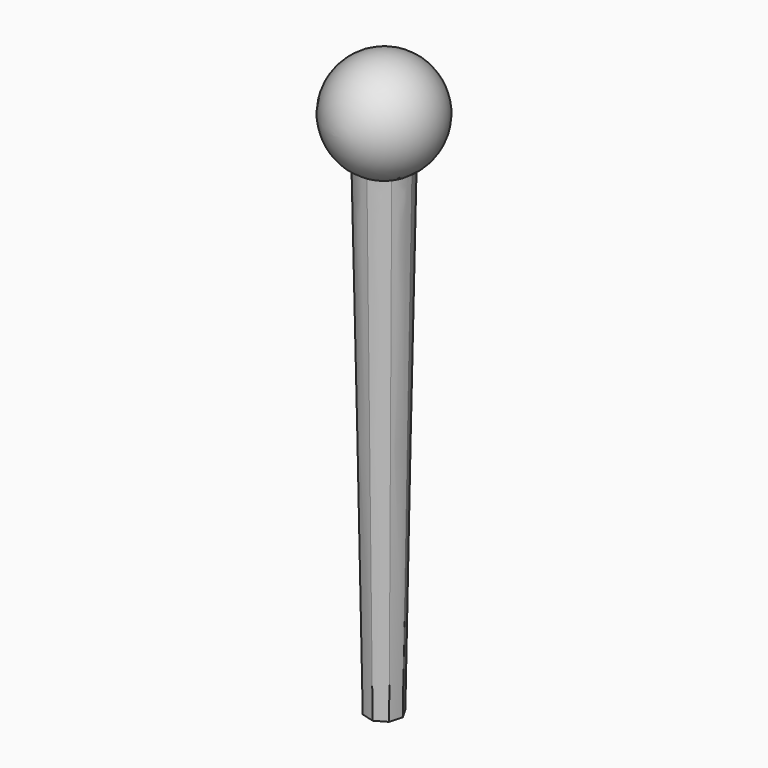
from build123d import *


# Not quite as in the source:
# - the arcs of a loft's sections are written as splines that run evenly, so that the points pair up as in the source's solid


with BuildPart() as f3:
    # F2 (on offset) → F3 section 0
    with BuildSketch(Plane.XY.offset(500)):
        with BuildLine():
            add(Edge.make_bspline(
                [(3.1036920521, -24.8065937937), (4.7272798193, -24.6034576239), (6.3308207683, -24.2404209935), (9.4363429336, -23.2084625424), (10.9382473598, -22.5395662389), (13.782772681, -20.9215792608), (15.1253232396, -19.972528594), (17.5995382038, -17.8306914211), (18.7311414296, -16.6379578761), (19.7355523864, -15.3462689929)],
                knots=[0, 0, 0, 0, 0.25, 0.25, 0.5, 0.5, 0.75, 0.75, 1, 1, 1, 1], degree=3))
            add(Edge.make_bspline(
                [(19.7355523864, -15.3462689929), (20.7399633433, -14.0545801097), (21.617132359, -12.6639997676), (23.0833633226, -9.7383591666), (23.6723890149, -8.2033712501), (24.5396825947, -5.0478985421), (24.8179290366, -3.427491776), (25.0529556268, -0.1634500075), (25.0097299635, 1.480104285), (24.8065937937, 3.1036920521)],
                knots=[0, 0, 0, 0, 0.25, 0.25, 0.5, 0.5, 0.75, 0.75, 1, 1, 1, 1], degree=3))
            add(Edge.make_bspline(
                [(24.8065937937, 3.1036920521), (24.6034576239, 4.7272798193), (24.2404209935, 6.3308207683), (23.2084625424, 9.4363429336), (22.5395662389, 10.9382473598), (20.9215792608, 13.782772681), (19.972528594, 15.1253232396), (17.8306914211, 17.5995382038), (16.6379578761, 18.7311414296), (15.3462689929, 19.7355523864)],
                knots=[0, 0, 0, 0, 0.25, 0.25, 0.5, 0.5, 0.75, 0.75, 1, 1, 1, 1], degree=3))
            add(Edge.make_bspline(
                [(15.3462689929, 19.7355523864), (14.0545801097, 20.7399633433), (12.6639997676, 21.617132359), (9.7383591666, 23.0833633226), (8.2033712501, 23.6723890149), (5.0478985421, 24.5396825947), (3.427491776, 24.8179290366), (0.1634500075, 25.0529556268), (-1.480104285, 25.0097299635), (-3.1036920521, 24.8065937937)],
                knots=[0, 0, 0, 0, 0.25, 0.25, 0.5, 0.5, 0.75, 0.75, 1, 1, 1, 1], degree=3))
            add(Edge.make_bspline(
                [(-3.1036920521, 24.8065937937), (-4.7272798193, 24.6034576239), (-6.3308207683, 24.2404209935), (-9.4363429336, 23.2084625424), (-10.9382473598, 22.5395662389), (-13.782772681, 20.9215792608), (-15.1253232396, 19.972528594), (-17.5995382038, 17.8306914211), (-18.7311414296, 16.6379578761), (-19.7355523864, 15.3462689929)],
                knots=[0, 0, 0, 0, 0.25, 0.25, 0.5, 0.5, 0.75, 0.75, 1, 1, 1, 1], degree=3))
            add(Edge.make_bspline(
                [(-19.7355523864, 15.3462689929), (-20.7399633433, 14.0545801097), (-21.617132359, 12.6639997676), (-23.0833633226, 9.7383591666), (-23.6723890149, 8.2033712501), (-24.5396825947, 5.0478985421), (-24.8179290366, 3.427491776), (-25.0529556268, 0.1634500075), (-25.0097299635, -1.480104285), (-24.8065937937, -3.1036920521)],
                knots=[0, 0, 0, 0, 0.25, 0.25, 0.5, 0.5, 0.75, 0.75, 1, 1, 1, 1], degree=3))
            add(Edge.make_bspline(
                [(-24.8065937937, -3.1036920521), (-24.6034576239, -4.7272798193), (-24.2404209935, -6.3308207683), (-23.2084625424, -9.4363429336), (-22.5395662389, -10.9382473598), (-20.9215792608, -13.782772681), (-19.972528594, -15.1253232396), (-17.8306914211, -17.5995382038), (-16.6379578761, -18.7311414296), (-15.3462689929, -19.7355523864)],
                knots=[0, 0, 0, 0, 0.25, 0.25, 0.5, 0.5, 0.75, 0.75, 1, 1, 1, 1], degree=3))
            add(Edge.make_bspline(
                [(-15.3462689929, -19.7355523864), (-14.0545801097, -20.7399633433), (-12.6639997676, -21.617132359), (-9.7383591666, -23.0833633226), (-8.2033712501, -23.6723890149), (-5.0478985421, -24.5396825947), (-3.427491776, -24.8179290366), (-0.1634500075, -25.0529556268), (1.480104285, -25.0097299635), (3.1036920521, -24.8065937937)],
                knots=[0, 0, 0, 0, 0.25, 0.25, 0.5, 0.5, 0.75, 0.75, 1, 1, 1, 1], degree=3))
        make_face()
    # F1 (on Top) → F3 section 1
    with BuildSketch(Plane.XY):
        Polygon((2.0156472416, -16.1102781829), (12.8169647829, -9.9664091169), (16.1102781829, 2.0156472416), (9.9664091169, 12.8169647829), (-2.0156472416, 16.1102781829), (-12.8169647829, 9.9664091169), (-16.1102781829, -2.0156472416), (-9.9664091169, -12.8169647829), align=None)
    loft(ruled=True)

    # F5 (on offset) → F6 (revolve)
    with BuildSketch(Plane.XY.offset(500)):
        with BuildLine():
            Line((0, -50), (0, 50))
            ThreePointArc((0, 50), (-50, 0), (0, -50))
        make_face()
    revolve(axis=Axis((0, 0, 500), (0, -1, 0)))


solid = f3.part
